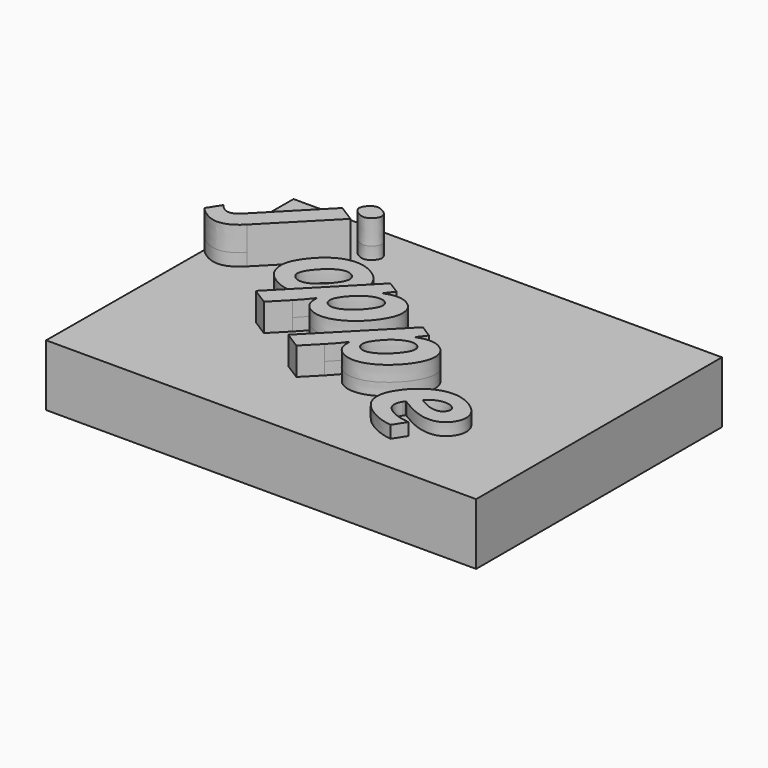
from build123d import *

# Parameters (mm, degrees)
F1_DEPTH     = 10
F2_TEXT_SIZE = 21.4429305338
F3_DEPTH     = 2
F4_DEPTH     = 4
F5_DEPTH     = 2.5


# Not quite as in the source:
# - Text() gives the source's letters only with a copy of the font that has no kerning and outlines rounded to 1/6400 em; it was checked with that copy


with BuildPart() as f1:
    # F0 (on Top) → F1 (new body)
    with BuildSketch(Plane.XY):
        Polygon((-34.8057380544, 20), (-35.0784632887, -30), (34.9215367113, -30), (34.9215367113, 20), align=None)
    extrude(amount=-F1_DEPTH)

    # F2 (on Top) → F3 (join)
    with BuildSketch(Plane.XY):
        with Locations(Location((-29.9429069747, 4.6443356455), (0, 0, -32.4832785763))):
            Text('joppe', F2_TEXT_SIZE, font='Open Sans', font_style=FontStyle.BOLDITALIC, text_align=(TextAlign.LEFT, TextAlign.BOTTOM))
    extrude(amount=F3_DEPTH)

    # F4 (add): faces of the model
    f4_faces = [f1.faces().sort_by_distance(p)[0] for p in [
        (-26.5526581598, 5.8101093077, 2),
        (-17.710910718, 14.3158337873, 2),
    ]]
    extrude(f4_faces, amount=F4_DEPTH)

    # F5 (add): faces of the model
    f5_faces = [f1.faces().sort_by_distance(p)[0] for p in [
        (-1.222812638, -6.723597189, 2),
        (9.5424604036, -13.5774164171, 2),
    ]]
    extrude(f5_faces, amount=F5_DEPTH)


solid = f1.part
